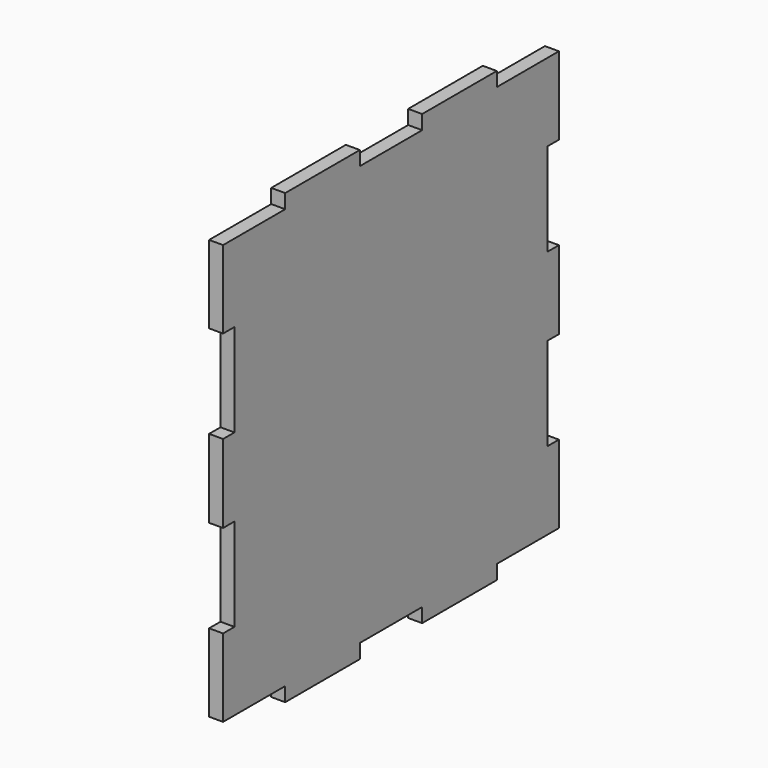
from build123d import *

# Parameters (mm, degrees)
F0_W     = 20
F0_H     = 3.05
F1_DEPTH = 3


# Not quite as in the source:
# - a feature names something its author has since deleted; it is built from what else it names


with BuildPart() as f1:
    # F0 (on Right) → F1 (new body)
    with BuildSketch(Plane.YZ):
        Polygon((28.35, -45), (45, -45), (45, -28.3), (41.95, -28.3), (41.95, -8.4), (45, -8.4), (45, 8.4), (41.95, 8.4), (41.95, 28.3), (45, 28.3), (45, 45), (28.35, 45), (8.35, 45), (-8.35, 45), (-28.35, 45), (-45, 45), (-45, 28.3), (-41.95, 28.3), (-41.95, 8.4), (-45, 8.4), (-45, -8.4), (-41.95, -8.4), (-41.95, -28.3), (-45, -28.3), (-45, -45), (-28.35, -45), (-8.35, -45), (8.35, -45), align=None)
        with Locations((-18.35, -46.525)):
            Rectangle(F0_W, F0_H)
        with Locations((18.35, -46.525)):
            Rectangle(F0_W, F0_H)
        with Locations((18.35, 46.525)):
            Rectangle(F0_W, F0_H)
        with Locations((-18.35, 46.525)):
            Rectangle(F0_W, F0_H)
    extrude(amount=F1_DEPTH)


solid = f1.part
